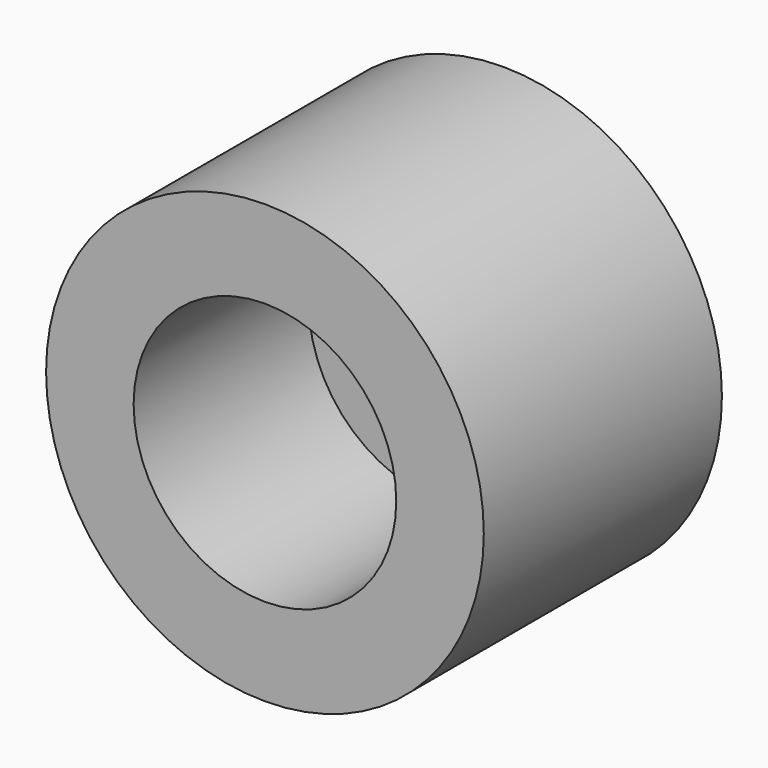
from build123d import *

# Parameters (mm, degrees)
F0_R     = 125
F0_R_2   = 75
F1_DEPTH = 150
F0_R_3   = 7.5
F0_R_4   = 10
F2_DEPTH = 25
F3_DEPTH = 150
F4_DEPTH = 20


with BuildPart() as f1:
    # F0 (on Front) → F1 (new body)
    with BuildSketch(Plane.XZ):
        Circle(F0_R)
        Circle(F0_R_2, mode=Mode.SUBTRACT)
    extrude(amount=F1_DEPTH)


with BuildPart() as f2:
    # F0 (on Front) → F2 (new body)
    with BuildSketch(Plane.XZ):
        Circle(F0_R_2)
        with Locations((-25, -25)):
            Circle(F0_R_3, mode=Mode.SUBTRACT)
        with Locations((25, -25)):
            Circle(F0_R_3, mode=Mode.SUBTRACT)
        with Locations((-25, 25)):
            Circle(F0_R_3, mode=Mode.SUBTRACT)
        Circle(F0_R_4, mode=Mode.SUBTRACT)
        with Locations((25, 25)):
            Circle(F0_R_3, mode=Mode.SUBTRACT)
    extrude(amount=F2_DEPTH)

    # F0 (on Front) → F3 (join)
    with BuildSketch(Plane.XZ):
        Circle(F0_R)
        Circle(F0_R_2, mode=Mode.SUBTRACT)
    extrude(amount=F3_DEPTH)

    # F0 (on Front) → F4 (join)
    with BuildSketch(Plane.XZ):
        Circle(F0_R)
        Circle(F0_R_2, mode=Mode.SUBTRACT)
    extrude(amount=-F4_DEPTH)


solid = Compound([f1.part, f2.part])
